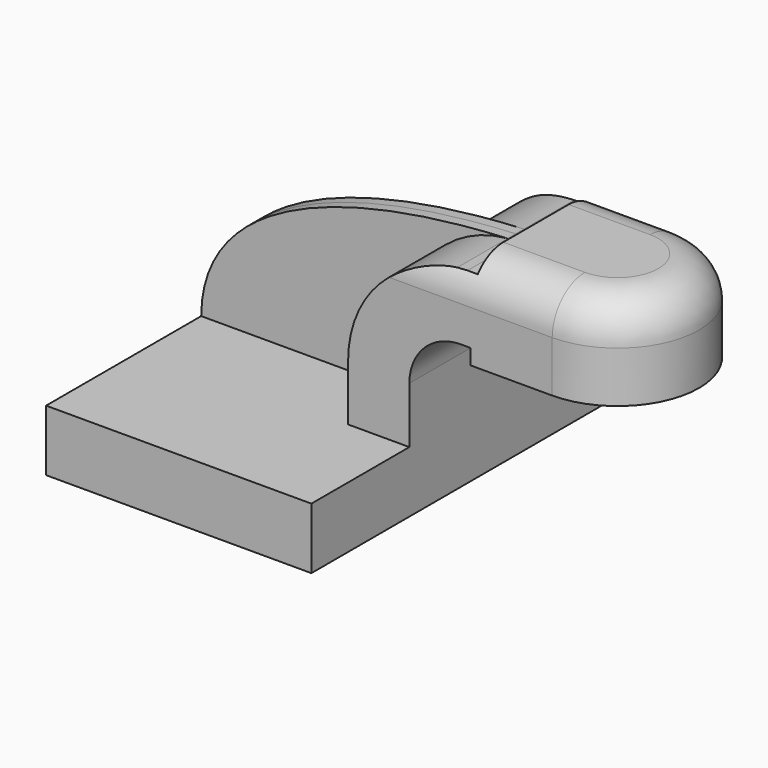
from build123d import *

# Parameters (mm, degrees)
F1_DEPTH = 63.5
F0_W     = 25.4
F0_H     = 19.05
F0_H_2   = 4.7498
F0_H_3   = 4.7752
F2_DEPTH = 25.4
F4_DEPTH = 3.175
F5_R     = 12.7


with BuildPart() as f1:
    # F0 (on Front) → F1 (new body, symmetric)
    with BuildSketch(Plane.XZ):
        Polygon((41.275, -9.525), (41.275, 9.525), (22.225, 9.525), (-41.275, 9.525), (-41.275, -9.525), align=None)
    extrude(amount=F1_DEPTH, both=True)

    # F0 (on Front) → F2 (join, symmetric)
    with BuildSketch(Plane.XZ):
        with BuildLine():
            Line((22.225, 9.525), (41.275, 9.525))
            Line((41.275, 9.525), (41.275, 27.0002))
            ThreePointArc((41.275, 27.0002), (45.9246798487, 38.2255201513), (57.15, 42.8752))
            Line((57.15, 42.8752), (60.325, 42.8752))
            Line((60.325, 42.8752), (60.325, 61.9252))
            Line((60.325, 61.9252), (57.15, 61.9252))
            add(Edge.make_bspline(
                [(54.0587441636, 61.7881255253), (55.0869767217, 61.838850256), (56.1175065912, 61.8845174455), (57.15, 61.9252)],
                knots=[109.2703067259, 109.2703067259, 109.2703067259, 109.2703067259, 111.5045361635, 111.5045361635, 111.5045361635, 111.5045361635], degree=3))
            ThreePointArc((54.0587441636, 61.7881255253), (31.3845411928, 50.5776629139), (22.225, 27.0002))
            Line((22.225, 27.0002), (22.225, 9.525))
        make_face()
        with Locations((73.025, 52.4002)):
            Rectangle(F0_W, F0_H)
        with Locations((73.025, 64.3001)):
            Rectangle(F0_W, F0_H_2)
        with Locations((73.025, 40.4876)):
            Rectangle(F0_W, F0_H_3)
    extrude(amount=F2_DEPTH, both=True)

    # F0 (on Front) → F3 (revolve)
    with BuildSketch(Plane.XZ):
        Polygon((85.725, 61.9252), (85.725, 42.8752), (85.725, 38.1), (111.125, 38.1), (111.125, 66.675), (85.725, 66.675), align=None)
    revolve(axis=Axis((85.725, 0, 52.3875), (0, 0, 1)))

    # F0 (on Front) → F4 (join, symmetric)
    with BuildSketch(Plane.XZ):
        with BuildLine():
            Line((-41.275, 9.525), (22.225, 9.525))
            Line((22.225, 9.525), (22.225, 27.0002))
            ThreePointArc((22.225, 27.0002), (31.3845411928, 50.5776629139), (54.0587441636, 61.7881255253))
            add(Edge.make_bspline(
                [(-41.275, 9.525), (-41.0225634855, 44.7292047169), (3.7705843511, 59.3073118764), (54.0587441636, 61.7881255253)],
                knots=[0, 0, 0, 0, 109.2703067259, 109.2703067259, 109.2703067259, 109.2703067259], degree=3))
        make_face()
    extrude(amount=F4_DEPTH, both=True)

    # F5
    f5_edges = [f1.edges().sort_by_distance(p)[0] for p in [
        (85.725, 25.4, 52.3875),
        (73.025, 25.4, 66.675),
        (73.025, -25.4, 66.675),
        (111.125, 0, 66.675),
    ]]
    fillet(f5_edges, radius=F5_R)


solid = f1.part
